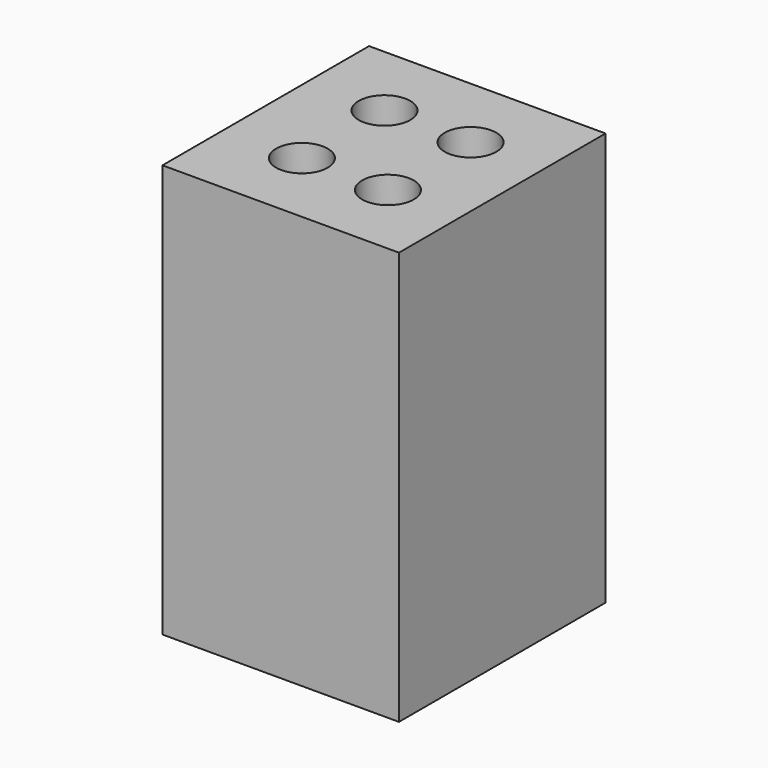
from build123d import *

# Parameters (mm, degrees)
F0_W     = 22.9004416908
F0_H     = 25
F0_R     = 2.5
F1_DEPTH = 40
F2_DEPTH = 40
F3_DEPTH = 5
F4_R     = 2.5


# Not quite as in the source:
# - a feature names something its author has since deleted; it is built from what else it names


with BuildPart() as f1:
    # F0 (on Top) → F1 (new body)
    with BuildSketch(Plane.XY):
        with Locations((-31.441590436, 3.4210662183)):
            Rectangle(F0_W, F0_H)
        with Locations((-35.3918112814, -1.5789337817)):
            Circle(F0_R, mode=Mode.SUBTRACT)
        with Locations((-27.0588112814, -1.5789337817)):
            Circle(F0_R, mode=Mode.SUBTRACT)
        with Locations((-35.3918112814, 8.4210662183)):
            Circle(F0_R, mode=Mode.SUBTRACT)
        with Locations((-27.0588112814, 8.4210662183)):
            Circle(F0_R, mode=Mode.SUBTRACT)
        with Locations((-35.3918112814, 8.4210662183)):
            Circle(F0_R)
        with Locations((-27.0588112814, 8.4210662183)):
            Circle(F0_R)
        with Locations((-27.0588112814, -1.5789337817)):
            Circle(F0_R)
        with Locations((-35.3918112814, -1.5789337817)):
            Circle(F0_R)
    extrude(amount=-F1_DEPTH)

    # F0 (on Top) → F2 (cut)
    with BuildSketch(Plane.XY):
        with Locations((-35.3918112814, 8.4210662183)):
            Circle(F0_R)
        with Locations((-27.0588112814, 8.4210662183)):
            Circle(F0_R)
    extrude(amount=-F2_DEPTH, mode=Mode.SUBTRACT)

    # F0 (on Top) → F3 (cut)
    with BuildSketch(Plane.XY):
        with Locations((-35.3918112814, -1.5789337817)):
            Circle(F0_R)
        with Locations((-27.0588112814, -1.5789337817)):
            Circle(F0_R)
    extrude(amount=-F3_DEPTH, mode=Mode.SUBTRACT)

    # F4
    f4_edges = [f1.edges().sort_by_distance(p)[0] for p in [
        (-37.891811, -1.578934, -5),
        (-29.558811, -1.578934, -5),
    ]]
    fillet(f4_edges, radius=F4_R)


solid = f1.part
